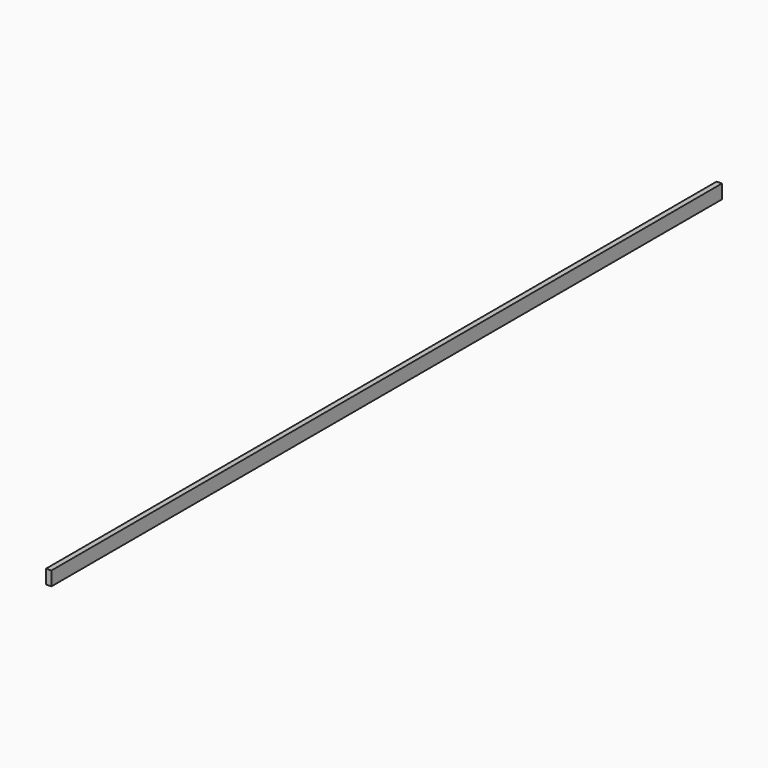
from build123d import *

# Parameters (mm, degrees)
F0_W     = 19.05
F0_H     = 50.8
F1_DEPTH = 3038.475


# Not quite as in the source:
# - a length typed as a fraction of an inch, garbled in the dataset ("3 / 203.2 mm" for 3/8 in), is restored


with BuildPart() as f1:
    # F0 (on Front) → F1 (new body)
    with BuildSketch(Plane.XZ):
        with Locations((9.525, -25.4)):
            Rectangle(F0_W, F0_H)
    extrude(amount=-F1_DEPTH)


solid = f1.part
